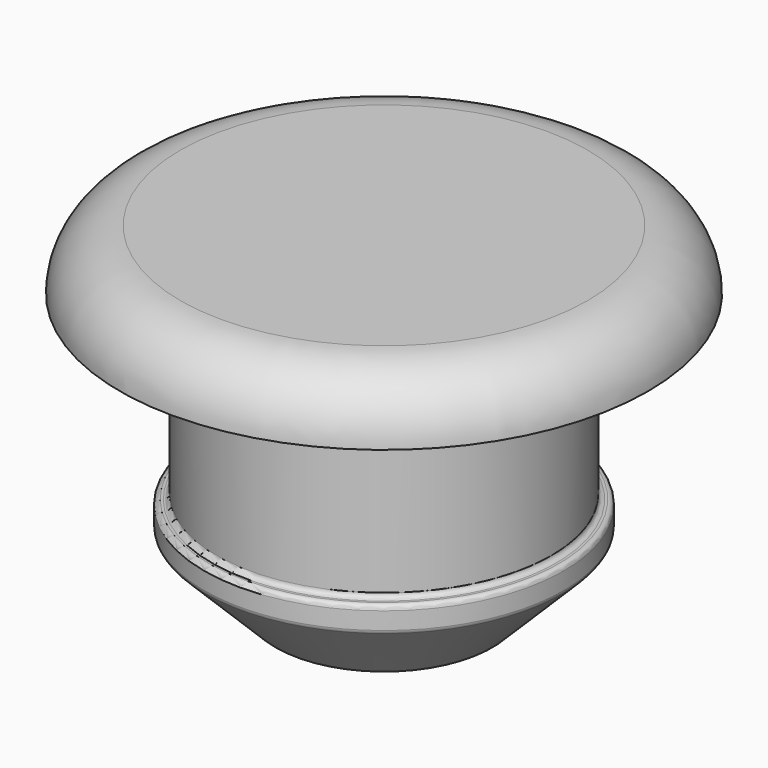
from build123d import *

# Parameters (mm, degrees)
F2_R    = 1.24999
F3_SIZE = 1.5
F4_R    = 0.1


# Not quite as in the source:
# - a fillet or chamfer is up to 0.001 mm smaller than in the source, because OpenCascade refuses the exact size


with BuildPart() as f1:
    # F0 (on Front) → F1 (revolve)
    with BuildSketch(Plane.XZ):
        Polygon((0, -7), (0, 0), (-5.475, 0), (-5.475, -1.25), (-3.475, -1.25), (-3.475, -5), (-3.725, -5), (-3.725, -7), align=None)
    revolve(axis=Axis((0, 0, -3.5), (0, 0, 1)))

    # F2 (radius 1.25 in the source; OpenCascade refuses exactly that, so slightly less here)
    f2_edges = [f1.edges().sort_by_distance(p)[0] for p in [
        (5.475, 0, 0),
    ]]
    fillet(f2_edges, radius=F2_R)

    # F3
    f3_edges = [f1.edges().sort_by_distance(p)[0] for p in [
        (3.725, 0, -7),
    ]]
    chamfer(f3_edges, length=F3_SIZE)

    # F4
    f4_edges = [f1.edges().sort_by_distance(p)[0] for p in [
        (3.725, 0, -5),
        (2.225, 0, -7),
        (3.475, 0, -5),
        (3.475, 0, -1.25),
        (3.725, 0, -5.5),
    ]]
    fillet(f4_edges, radius=F4_R)


solid = f1.part
